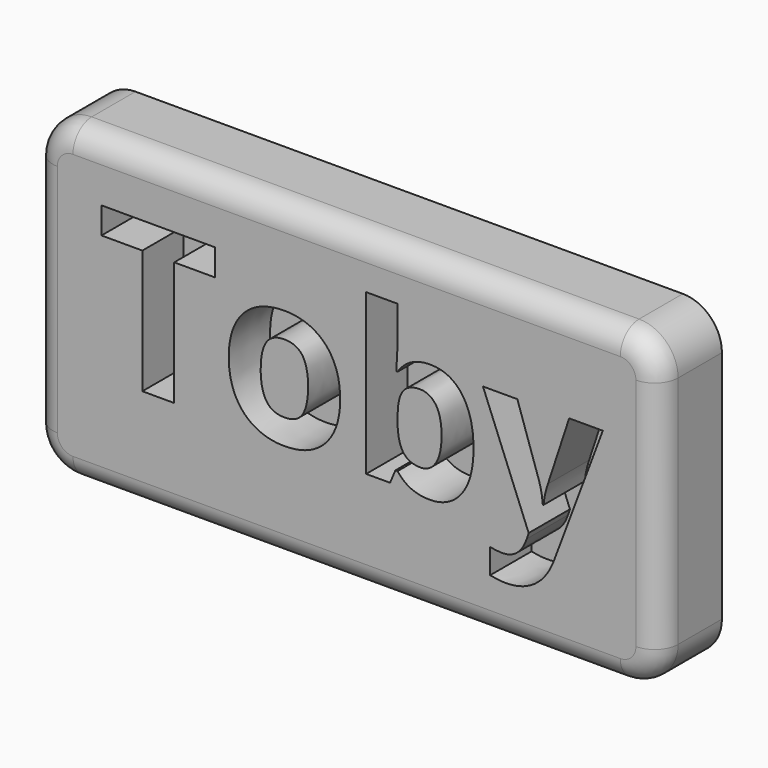
from build123d import *

# Parameters (mm, degrees)
F0_W         = 40
F0_H         = 20
F1_DEPTH     = 5
F2_R         = 2.5
F3_R         = 1.5
F4_TEXT_SIZE = 13.4698276977
F5_DEPTH     = 3.3


# Not quite as in the source:
# - Text() gives the source's letters only with a copy of the font that has no kerning and outlines rounded to 1/6400 em; it was checked with that copy


with BuildPart() as f1:
    # F0 (on Front) → F1 (new body)
    with BuildSketch(Plane.XZ):
        Rectangle(F0_W, F0_H)
    extrude(amount=F1_DEPTH)

    # F2
    f2_edges = [f1.edges().sort_by_distance(p)[0] for p in [
        (-20, -2.5, 10),
        (-20, -2.5, -10),
        (20, -2.5, 10),
        (20, -2.5, -10),
    ]]
    fillet(f2_edges, radius=F2_R)

    # F3
    f3_edges = [f1.edges().sort_by_distance(p)[0] for p in [
        (0, -5, 10),
    ]]
    fillet(f3_edges, radius=F3_R)

    # F4 (on face) → F5 (cut)
    with BuildSketch(Plane.XZ.offset(5)):
        with Locations((-15.944218263, -3.3927699551)):
            Text('Toby', F4_TEXT_SIZE, font='Open Sans', font_style=FontStyle.BOLD, text_align=(TextAlign.LEFT, TextAlign.BOTTOM))
    extrude(amount=-F5_DEPTH, mode=Mode.SUBTRACT)


solid = f1.part
